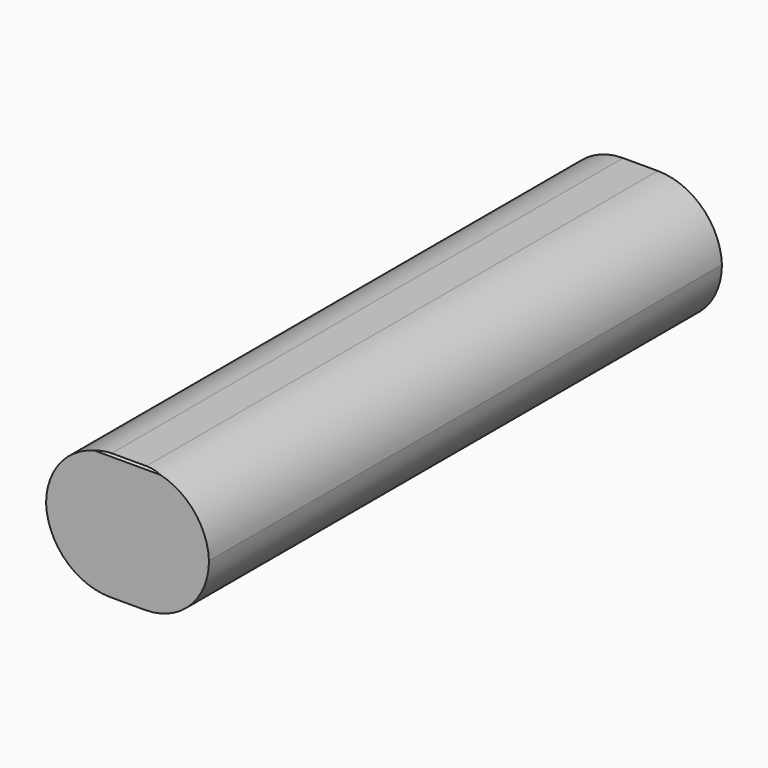
from build123d import *

# Parameters (mm, degrees)
F0_W          = 64.5265355706
F0_H          = 49.8596951365
F1_DEPTH      = 127
F1_DEPTH_BACK = 127
F3_T1_DEPTH   = 68.4457804443
F4_R          = 25.4
F5_T1_DEPTH   = 380.9129452384
F7_T1_DEPTH   = 380.1509452384


# Not quite as in the source:
# - a fillet or chamfer that OpenCascade refuses, or shapes differently, is made with other operations: its cross-section is extruded or revolved along the edge and cut away or added
# - two fillets or chamfers of one size are made in one step
# - a feature of the source that left no trace in its solid (it failed there, or was rolled back) is left out


with BuildPart() as f1:
    # F0 (on Front) → F1 (new body, two sides)
    with BuildSketch(Plane.XZ) as f1_sk:
        with Locations((-32.2632677853, 24.9298475683)):
            Rectangle(F0_W, F0_H)
    extrude(amount=F1_DEPTH)
    extrude(f1_sk.sketch, amount=-F1_DEPTH_BACK)

    # F3: chamfer of 0.762 on 1 edges, made by hand

    # F3_s2 → F3_t1 (cut)
    with BuildSketch(Plane.YZ.offset(-66.4861580075)):
        Polygon((-126.238, 49.8596951365), (-127, 49.0976951365), (-127, 49.8596951365), align=None)
    extrude(amount=F3_T1_DEPTH, mode=Mode.SUBTRACT)

    # F4
    f4_edges = [f1.edges().sort_by_distance(p)[0] for p in [
        (-64.526536, 0.381, 49.859695),
        (0, 0, 0),
    ]]
    fillet(f4_edges, radius=F4_R)

    # F5: fillet of radius 25.4 on 1 edges, made by hand

    # F5_s2 → F5_t1 (cut)
    with BuildSketch(Plane.XZ.offset(-190.4564726192)):
        with BuildLine():
            ThreePointArc((-64.5265355706, 24.4596951365), (-56.7688756926, 7.1100609141), (-39.1439465229, 0))
            Line((-39.1439465229, 0), (-64.5265355706, 0))
            Line((-64.5265355706, 0), (-64.5265355706, 24.4596951365))
        make_face()
    extrude(amount=F5_T1_DEPTH, mode=Mode.SUBTRACT)

    # F7: fillet of radius 25.4 on 1 edges, made by hand

    # F7_s2 → F7_t1 (cut)
    with BuildSketch(Plane.XZ.offset(-190.4564726192)):
        with BuildLine():
            ThreePointArc((-25.3825890477, 49.8596951365), (-7.7576598781, 42.7496342224), (0, 25.4))
            Line((0, 25.4), (0, 49.8596951365))
            Line((0, 49.8596951365), (-25.3825890477, 49.8596951365))
        make_face()
    extrude(amount=F7_T1_DEPTH, mode=Mode.SUBTRACT)


solid = f1.part
